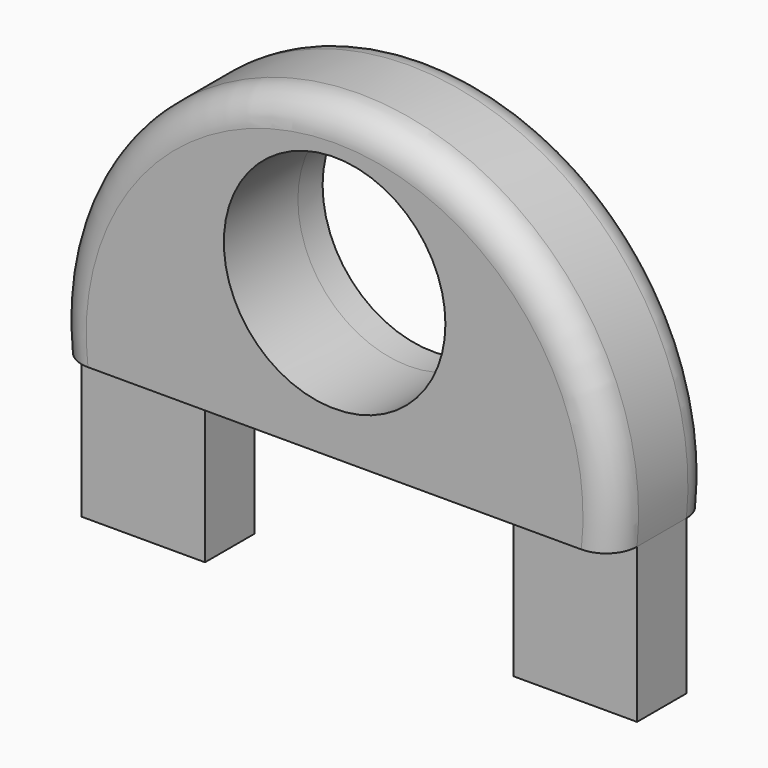
from build123d import *
from build123d import SkipClean  # not in build123d's __all__

# Parameters (mm, degrees)
F0_R        = 3.59
F1_DEPTH    = 2
F2_R        = 3.59
F3_DEPTH    = 1
F4_R        = 3.59
F5_DEPTH    = 1
F7_T3_ANGLE = 223.7642380541
F7_T6_ANGLE = 223.7642380541


# Not quite as in the source:
# - a fillet or chamfer that OpenCascade refuses, or shapes differently, is made with other operations: its cross-section is extruded or revolved along the edge and cut away or added
# - a feature of the source that left no trace in its solid (it failed there, or was rolled back) is left out


with BuildPart() as f1:
    # F0 (on Front) → F1 (new body)
    with BuildSketch(Plane.XZ):
        with BuildLine():
            Line((-28.8239947557, 12.7150369808), (-28.8239947557, 17.7150369808))
            Line((-28.8239947557, 17.7150369808), (-18.8239947557, 17.7150369808))
            Line((-18.8239947557, 17.7150369808), (-18.8239947557, 12.7150369808))
            Line((-18.8239947557, 12.7150369808), (-14.8239947557, 12.7150369808))
            Line((-14.8239947557, 12.7150369808), (-14.8239947557, 17.7150369808))
            ThreePointArc((-14.8239947557, 17.7150369808), (-23.8239947557, 27.7150369808), (-32.8239947557, 17.7150369808))
            Line((-32.8239947557, 17.7150369808), (-32.8239947557, 12.7150369808))
            Line((-32.8239947557, 12.7150369808), (-28.8239947557, 12.7150369808))
        make_face()
        with Locations((-23.8239947557, 22.7150369808)):
            Circle(F0_R, mode=Mode.SUBTRACT)
    extrude(amount=F1_DEPTH)

    # F2 (on face) → F3 (join)
    with BuildSketch(Plane.XZ.offset(2)):
        with BuildLine():
            Line((-32.8239947557, 17.7150369808), (-28.8239947557, 17.7150369808))
            Line((-28.8239947557, 17.7150369808), (-18.8239947557, 17.7150369808))
            Line((-18.8239947557, 17.7150369808), (-14.8239947557, 17.7150369808))
            ThreePointArc((-14.8239947557, 17.7150369808), (-23.8239947557, 27.7150369808), (-32.8239947557, 17.7150369808))
        make_face()
        with Locations((-23.8239947557, 22.7150369808)):
            Circle(F2_R, mode=Mode.SUBTRACT)
    extrude(amount=F3_DEPTH)

    # F4 (on face) → F5 (join)
    with BuildSketch(Plane(origin=(0, 0, 0), x_dir=(-1, 0, 0), z_dir=(0, 1, 0))):
        with BuildLine():
            Line((14.8239947557, 17.7150369808), (18.8239947557, 17.7150369808))
            Line((18.8239947557, 17.7150369808), (28.8239947557, 17.7150369808))
            Line((28.8239947557, 17.7150369808), (32.8239947557, 17.7150369808))
            ThreePointArc((32.8239947557, 17.7150369808), (23.8239947557, 27.7150369808), (14.8239947557, 17.7150369808))
        make_face()
        with Locations((23.8239947557, 22.7150369808)):
            Circle(F4_R, mode=Mode.SUBTRACT)
    with SkipClean():  # cleaning this boolean's faces spoils the solid; the shape is the same uncleaned
        extrude(amount=F5_DEPTH)

    # F7: fillet of radius 1 on 2 edges, made by hand


with BuildPart() as f7_tool1:
    # F7_s2 → F7_t3 (revolve)
    with BuildSketch(Plane(origin=(3.1459864442, 0, 7.8329498468), x_dir=(0, 1, 0), z_dir=(-0.3726982036, 0, -0.9279526114))):
        with BuildLine():
            ThreePointArc((-2, -20.0139639005), (-2.7071067812, -20.3068571193), (-3, -21.0139639005))
            Line((-3, -21.0139639005), (-3, -20.0139639005))
            Line((-3, -20.0139639005), (-2, -20.0139639005))
        make_face()
    revolve(axis=Axis((-23.8239947557, -3, 18.6650369808), (0, -1, 0)), revolution_arc=F7_T3_ANGLE)


with BuildPart() as f7_tool4:
    # F7_s5 → F7_t6 (revolve)
    with BuildSketch(Plane(origin=(-9.7644804416, 0, 24.3118293528), x_dir=(0, 1, 0), z_dir=(0.3726982036, 0, -0.9279526114))):
        with BuildLine():
            ThreePointArc((0, -24.2011123962), (0.7071067812, -23.9082191774), (1, -23.2011123962))
            Line((1, -23.2011123962), (1, -24.2011123962))
            Line((1, -24.2011123962), (0, -24.2011123962))
        make_face()
    revolve(axis=Axis((-23.8239947557, 1, 18.6650369808), (0, 1, 0)), revolution_arc=F7_T6_ANGLE)


with BuildPart() as f1_1:
    add(f1.part, clean=False)

    # F7_t7: cut F7_tool1, F7_tool4
    add([f7_tool1.part, f7_tool4.part], mode=Mode.SUBTRACT)


solid = f1_1.part
